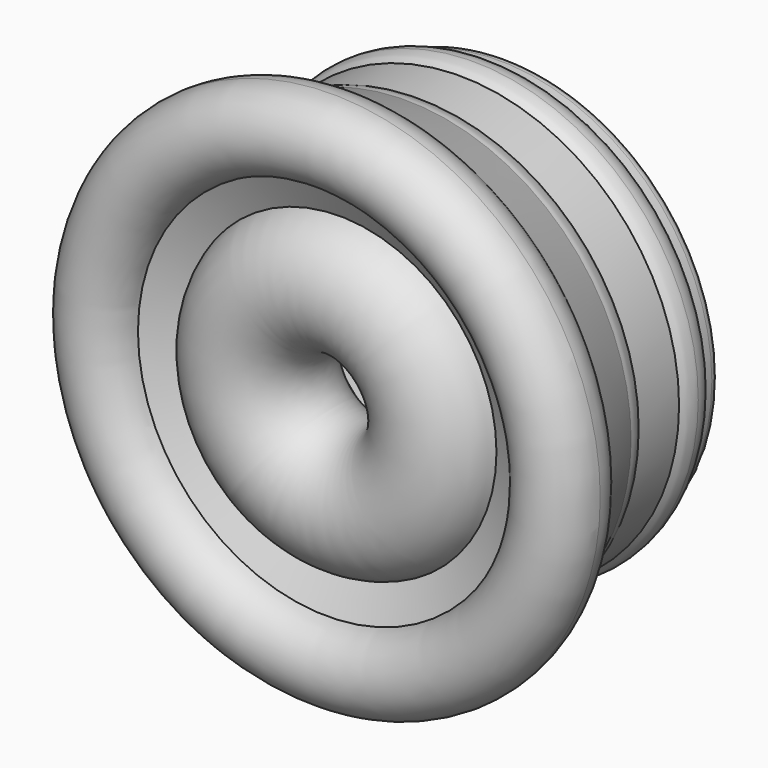
from build123d import *

# Parameters (mm, degrees)
F2_R = 5.08
F3_R = 5.08


with BuildPart() as f1:
    # F0 (on Top) → F1 (revolve)
    with BuildSketch(Plane.XY):
        with BuildLine():
            ThreePointArc((9.7009118807, 40.9040962808), (11.7520070447, 44.5794186576), (12.4627258003, 48.7278960645))
            ThreePointArc((12.4627258003, 48.7278960645), (11.0166338716, 54.5548431652), (7.0139478912, 59.0295497839))
            ThreePointArc((7.0139478912, 59.0295497839), (1.7832953622, 61.0623758681), (-3.8089326117, 60.594301027))
            ThreePointArc((-3.8089326117, 60.594301027), (-10.5985925253, 55.2845240741), (-12.3186808909, 46.8385481656))
            ThreePointArc((-12.3186808909, 46.8385481656), (-11.2979086397, 43.4670221122), (-9.3744965448, 40.5158105252))
            ThreePointArc((-9.3744965448, 40.5158105252), (-1.9976894845, 36.4263201046), (6.2941219653, 37.971336993))
            ThreePointArc((6.2941219653, 37.971336993), (8.130839206, 39.2828450758), (9.7009118807, 40.9040962808))
        make_face()
        with BuildLine():
            ThreePointArc((-3.8089326117, 60.594301027), (1.7832953622, 61.0623758681), (7.0139478912, 59.0295497839))
            Line((7.0139478912, 59.0295497839), (7.0139478912, 68.5800015926))
            Line((7.0139478912, 68.5800015926), (-3.8089326117, 68.5800015926))
            Line((-3.8089326117, 68.5800015926), (-3.8089326117, 60.594301027))
        make_face()
        with BuildLine():
            Line((9.7009118807, 17.1683712151), (9.7009118807, 40.9040962808))
            ThreePointArc((9.7009118807, 40.9040962808), (8.130839206, 39.2828450758), (6.2941219653, 37.971336993))
            Line((6.2941219653, 37.971336993), (6.2941219653, 20.0158471298))
            ThreePointArc((6.2941219653, 20.0158471298), (8.1232571488, 18.7425478578), (9.7009118807, 17.1683712151))
        make_face()
        with BuildLine():
            Line((6.2941219653, 20.0158471298), (6.2941219653, 37.971336993))
            ThreePointArc((6.2941219653, 37.971336993), (-1.9976894845, 36.4263201046), (-9.3744965448, 40.5158105252))
            Line((-9.3744965448, 40.5158105252), (-42.5554838048, 7.7026077091))
            ThreePointArc((-42.5554838048, 7.7026077091), (-34.4707888035, 4.93903315), (-27.4990179272, 0))
            Line((-27.4990179272, 0), (-12.0346660983, 5.0726801795))
            ThreePointArc((-12.0346660983, 5.0726801795), (-8.003937866, 18.8410461734), (6.2941219653, 20.0158471298))
        make_face()
        with BuildLine():
            ThreePointArc((12.6666341186, 9.023684077), (11.9021326094, 13.3576036935), (9.7009118807, 17.1683712151))
            ThreePointArc((9.7009118807, 17.1683712151), (8.1232571488, 18.7425478578), (6.2941219653, 20.0158471298))
            ThreePointArc((6.2941219653, 20.0158471298), (-8.003937866, 18.8410461734), (-12.0346660983, 5.0726801795))
            ThreePointArc((-12.0346660983, 5.0726801795), (-10.7649616155, 2.3484146958), (-8.8891363795, 0))
            ThreePointArc((-8.8891363795, 0), (4.8787983734, -2.6656677582), (12.666605472, 8.996745052))
            ThreePointArc((12.666605472, 8.996745052), (12.666626957, 9.0102145568), (12.6666341186, 9.023684077))
        make_face()
        with BuildLine():
            ThreePointArc((-9.3744965448, 40.5158105252), (-11.2979086397, 43.4670221122), (-12.3186808909, 46.8385481656))
            Line((-12.3186808909, 46.8385481656), (-52.7847993644, 7.8438725712))
            ThreePointArc((-52.7847993644, 7.8438725712), (-47.6640495586, 8.2143778422), (-42.5554838048, 7.7026077091))
            Line((-42.5554838048, 7.7026077091), (-9.3744965448, 40.5158105252))
        make_face()
        with BuildLine():
            ThreePointArc((-42.5554838048, 7.7026077091), (-47.6640495586, 8.2143778422), (-52.7847993644, 7.8438725712))
            ThreePointArc((-52.7847993644, 7.8438725712), (-70.4822634568, -41.4156089372), (-19.396468474, -30.0165605224))
            ThreePointArc((-19.396468474, -30.0165605224), (-18.5027603086, -25.8789123067), (-18.2028503372, -21.656483971))
            ThreePointArc((-18.2028503372, -21.656483971), (-18.3038042539, -19.2026004419), (-18.6059836854, -16.7653020075))
            ThreePointArc((-18.6059836854, -16.7653020075), (-20.3241438407, -10.6001768173), (-23.3160750285, -4.9425102755))
            ThreePointArc((-23.3160750285, -4.9425102755), (-25.2732427868, -2.3575913031), (-27.4990179272, 0))
            ThreePointArc((-27.4990179272, 0), (-34.4707888035, 4.93903315), (-42.5554838048, 7.7026077091))
        make_face()
        with BuildLine():
            ThreePointArc((-8.8891363795, 0), (-10.7649616155, 2.3484146958), (-12.0346660983, 5.0726801795))
            Line((-12.0346660983, 5.0726801795), (-27.4990179272, 0))
            ThreePointArc((-27.4990179272, 0), (-25.2732427868, -2.3575913031), (-23.3160750285, -4.9425102755))
            Line((-23.3160750285, -4.9425102755), (-8.8891363795, 0))
        make_face()
        with BuildLine():
            Line((24.0191616365, -18.4949137387), (12.666605472, 8.996745052))
            ThreePointArc((12.666605472, 8.996745052), (4.8787983734, -2.6656677582), (-8.8891363795, 0))
            Line((-8.8891363795, 0), (-23.3160750285, -4.9425102755))
            ThreePointArc((-23.3160750285, -4.9425102755), (-20.3241438407, -10.6001768173), (-18.6059836854, -16.7653020075))
            Line((-18.6059836854, -16.7653020075), (-2.9157078566, -26.9645396174))
            ThreePointArc((-2.9157078566, -26.9645396174), (5.888669157, -17.6376063496), (18.6366916792, -16.224573954))
            ThreePointArc((18.6366916792, -16.224573954), (21.4175881123, -17.1471765082), (24.0191616365, -18.4949137387))
        make_face()
        with BuildLine():
            ThreePointArc((-18.2028503372, -21.656483971), (-18.5027603086, -25.8789123067), (-19.396468474, -30.0165605224))
            Line((-19.396468474, -30.0165605224), (-4.1937379558, -37.1727543587))
            ThreePointArc((-4.1937379558, -37.1727543587), (-4.274336975, -31.9785540126), (-2.9157078566, -26.9645396174))
            Line((-2.9157078566, -26.9645396174), (-18.6059836854, -16.7653020075))
            ThreePointArc((-18.6059836854, -16.7653020075), (-18.3038042539, -19.2026004419), (-18.2028503372, -21.656483971))
        make_face()
        with BuildLine():
            ThreePointArc((32.792011574, -34.2898162166), (30.4515944815, -25.2559654275), (24.0191616365, -18.4949137387))
            ThreePointArc((24.0191616365, -18.4949137387), (21.4175881123, -17.1471765082), (18.6366916792, -16.224573954))
            ThreePointArc((18.6366916792, -16.224573954), (5.888669157, -17.6376063496), (-2.9157078566, -26.9645396174))
            ThreePointArc((-2.9157078566, -26.9645396174), (-4.274336975, -31.9785540126), (-4.1937379558, -37.1727543587))
            ThreePointArc((-4.1937379558, -37.1727543587), (15.6326196944, -52.8387851947), (32.792011574, -34.2898162166))
        make_face()
    revolve(axis=Axis((-93.19460392, 9.023681283, 0), (0, -1, 0)))

    # F2
    f2_edges = [f1.edges().sort_by_distance(p)[0] for p in [
        (-193.403156, 68.580002, 0),
    ]]
    fillet(f2_edges, radius=F2_R)

    # F3
    f3_edges = [f1.edges().sort_by_distance(p)[0] for p in [
        (-210.408369, -18.494914, 0),
    ]]
    fillet(f3_edges, radius=F3_R)


solid = f1.part
